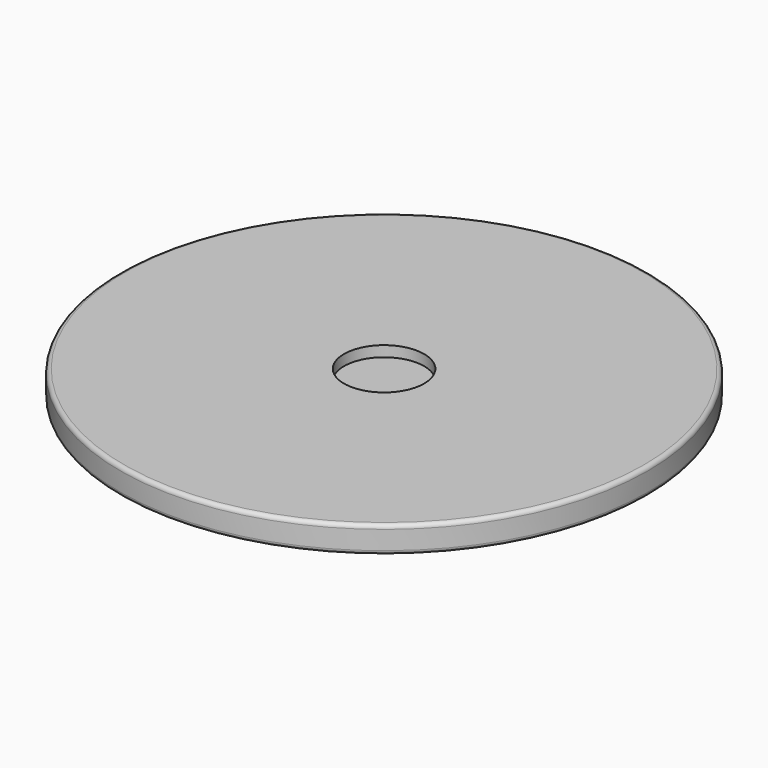
from build123d import *

# Parameters (mm, degrees)
F0_R     = 9.885
F1_DEPTH = 1
F2_R     = 0.15
F3_R     = 1.5
F4_DEPTH = 0.4


# Not quite as in the source:
# - a feature names something its author has since deleted; it is built from what else it names


with BuildPart() as f1:
    # F0 (on Top) → F1 (new body)
    with BuildSketch(Plane.XY):
        Circle(F0_R)
    extrude(amount=F1_DEPTH)

    # F2
    f2_edges = [f1.edges().sort_by_distance(p)[0] for p in [
        (-9.885, 0, 1),
        (-9.885, 0, 0),
    ]]
    fillet(f2_edges, radius=F2_R)

    # F3 (on face) → F4 (cut)
    with BuildSketch(Plane.XY.offset(1)):
        Circle(F3_R)
    extrude(amount=-F4_DEPTH, mode=Mode.SUBTRACT)


solid = f1.part
